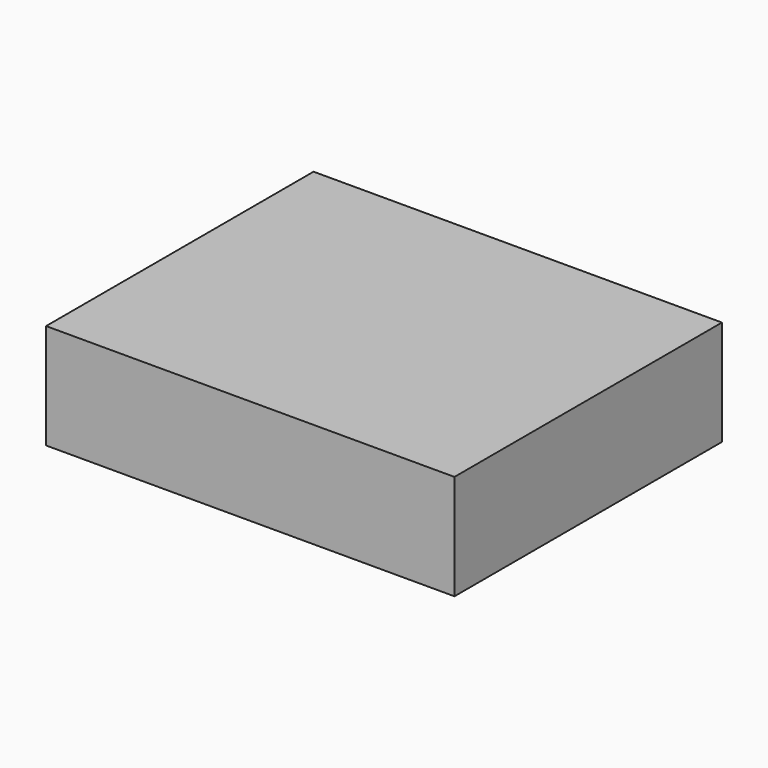
from build123d import *

# Parameters (mm, degrees)
F0_W     = 137.9
F0_H     = 112.9
F1_DEPTH = 35.5


# Not quite as in the source:
# - the program builds the solid bodies; features that only make, move or delete a surface that nothing else refers to are left out


with BuildPart() as f1:
    # F0 (on Top) → F1 (new body)
    with BuildSketch(Plane.XY):
        with Locations((46.9436596751, 27.8300400496)):
            Rectangle(F0_W, F0_H)
    extrude(amount=F1_DEPTH)


solid = f1.part
